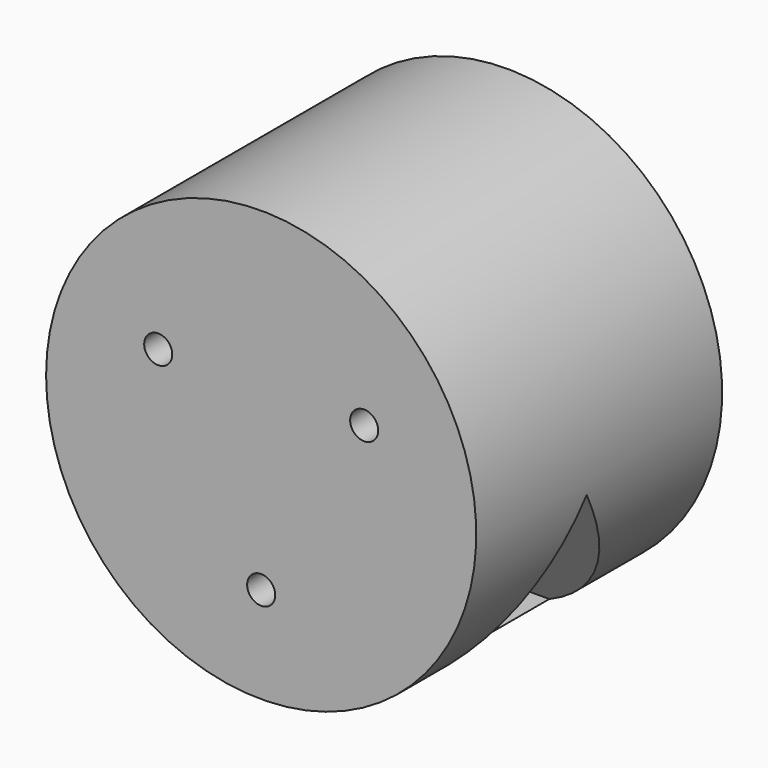
from build123d import *

# Parameters (mm, degrees)
F0_W          = 51.8020391464
F0_H          = 74.018985033
F3_D          = 6.7564
F5_DEPTH      = 51.8030391464
F5_DEPTH_BACK = 51.8030391464


with BuildPart() as f1:
    # F0 (on Top) → F1 (revolve)
    with BuildSketch(Plane.XY):
        with Locations((-25.9010195732, 3.415748477)):
            Rectangle(F0_W, F0_H)
    revolve(axis=Axis((0, 3.415748477, 0), (0, -1, 0)))

    # F3 (through all)
    with Locations(Plane(origin=(0, 40.4252409935, 0), x_dir=(-1, 0, 0), z_dir=(0, 1, 0))):
        with Locations((-24.7987365379, 14.3175572157), (0, -28.6351144314), (24.7987365379, 14.3175572157)):
            Hole(F3_D / 2)

    # F4 (on Right) → F5 (cut, two sides)
    with BuildSketch(Plane.YZ) as f5_sk:
        Polygon((-23.4744153275, -46.0438393056), (23.4744153275, -46.0438393056), (0, -5.3849592805), align=None)
    extrude(amount=F5_DEPTH, mode=Mode.SUBTRACT)
    extrude(f5_sk.sketch, amount=-F5_DEPTH_BACK, mode=Mode.SUBTRACT)


solid = f1.part
